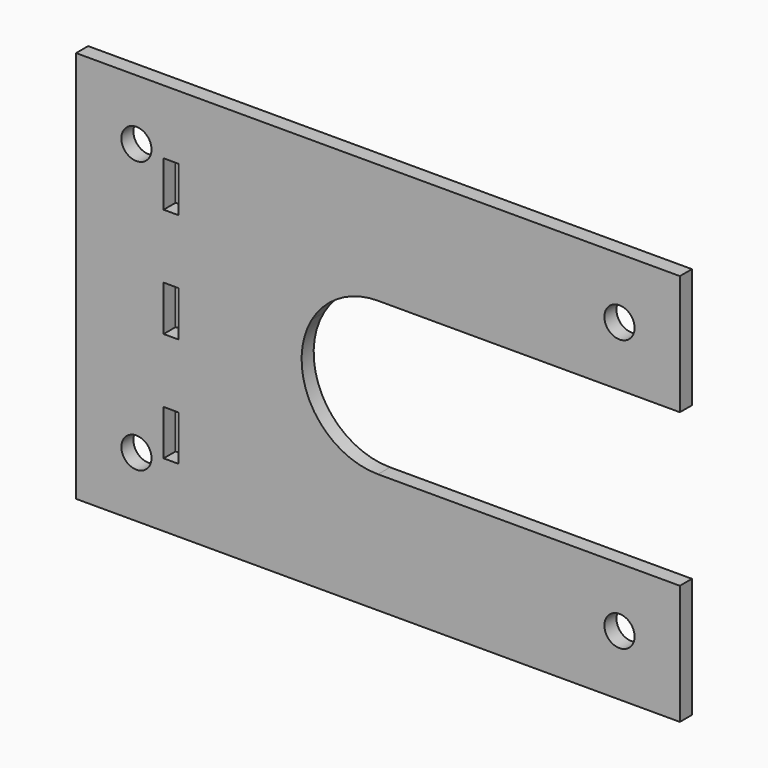
from build123d import *

# Parameters (mm, degrees)
F0_R     = 5
F0_W     = 5
F0_H     = 15
F0_W_2   = 40
F0_H_2   = 8
F1_DEPTH = 5


# Not quite as in the source:
# - a feature names something its author has since deleted; it is built from what else it names


with BuildPart() as f1:
    # F0 (on Front) → F1 (new body)
    with BuildSketch(Plane.XZ):
        with BuildLine():
            Line((0, 122), (0, 0))
            Line((0, 0), (40, 0))
            Line((40, 0), (42, 0))
            Line((42, 0), (158, 0))
            Line((158, 0), (160, 0))
            Line((160, 0), (200, 0))
            Line((200, 0), (200, 39.7))
            Line((200, 39.7), (159.7, 39.7))
            Line((159.7, 39.7), (143.1136062057, 39.7))
            ThreePointArc((143.1136062057, 39.7), (138.9711431703, 37.5), (134.8286801349, 39.7))
            Line((134.8286801349, 39.7), (100, 39.7))
            ThreePointArc((100, 39.7), (78.0895572843, 52.35), (78.0895572843, 77.65))
            ThreePointArc((78.0895572843, 77.65), (87.35, 86.9104427157), (100, 90.3))
            Line((100, 90.3), (159.7, 90.3))
            Line((159.7, 90.3), (200, 90.3))
            Line((200, 90.3), (200, 122))
            Line((200, 122), (160, 122))
            Line((160, 122), (158, 130))
            Line((158, 130), (42, 130))
            Line((42, 130), (40, 122))
            Line((40, 122), (0, 122))
        make_face()
        with Locations((20, 20)):
            Circle(F0_R, mode=Mode.SUBTRACT)
        with Locations((31.5, 28.75)):
            Rectangle(F0_W, F0_H, mode=Mode.SUBTRACT)
        with Locations((180, 20)):
            Circle(F0_R, mode=Mode.SUBTRACT)
        with Locations((31.5, 65)):
            Rectangle(F0_W, F0_H, mode=Mode.SUBTRACT)
        with BuildLine():
            ThreePointArc((66.0288568297, 87.5), (65.8584859611, 86.2059047745), (65.3589838486, 85))
            ThreePointArc((65.3589838486, 85), (56.1992276983, 88.7940952255), (66.0288568297, 87.5))
        make_face(mode=Mode.SUBTRACT)
        with Locations((20, 110)):
            Circle(F0_R, mode=Mode.SUBTRACT)
        with Locations((31.5, 101.25)):
            Rectangle(F0_W, F0_H, mode=Mode.SUBTRACT)
        with Locations((180, 110)):
            Circle(F0_R, mode=Mode.SUBTRACT)
        with BuildLine():
            ThreePointArc((66.0288568297, 87.5), (56.1992276983, 88.7940952255), (65.3589838486, 85))
            ThreePointArc((65.3589838486, 85), (65.8584859611, 86.2059047745), (66.0288568297, 87.5))
        make_face()
        with Locations((20, 126)):
            Rectangle(F0_W_2, F0_H_2)
        with Locations((180, 126)):
            Rectangle(F0_W_2, F0_H_2)
        Polygon((160, 130), (158, 130), (160, 122), align=None)
        Polygon((40, 130), (40, 122), (42, 130), align=None)
        with BuildLine():
            ThreePointArc((134.8286801349, 39.7), (138.9711431703, 37.5), (143.1136062057, 39.7))
            Line((143.1136062057, 39.7), (134.8286801349, 39.7))
        make_face()
    extrude(amount=F1_DEPTH)


solid = f1.part
